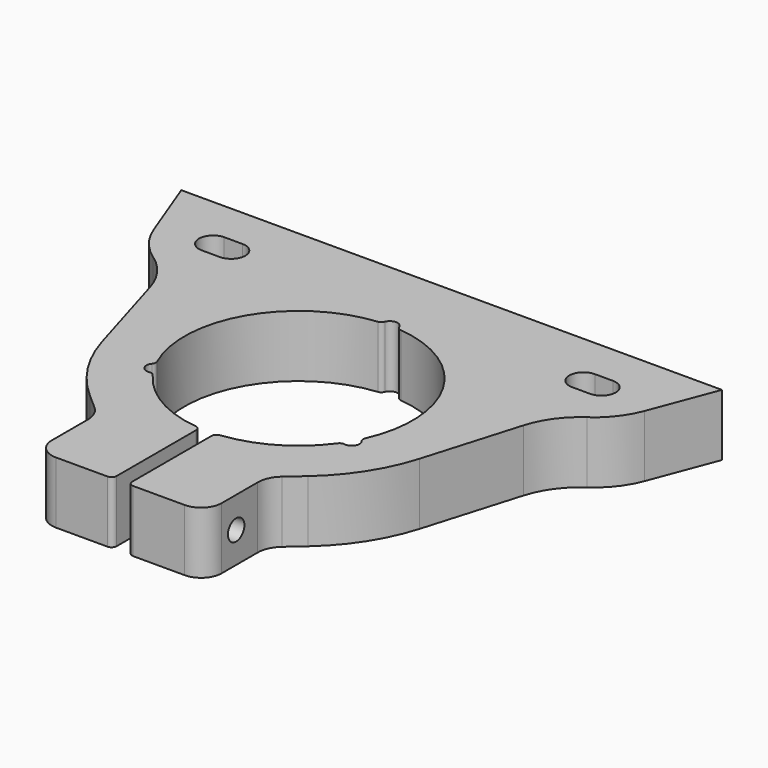
from build123d import *

# Parameters (mm, degrees)
F1_DEPTH = 12
F2_R     = 5
F3_R     = 2
F4_DEPTH = 69.001
F5_R     = 4
F6_R     = 2
F7_DEPTH = 12
F8_R     = 1.5
F9_DEPTH = 25
F10_R    = 1


with BuildPart() as f1:
    # F0 (on Top) → F1 (new body)
    with BuildSketch(Plane.XY):
        with BuildLine():
            Line((52.5, 0), (-52.5, 0))
            Line((-52.5, 0), (-47.6682177495, -12.7529115916))
            ThreePointArc((-47.6682177495, -12.7529115916), (-45.4487126417, -16.689553935), (-42.1574376197, -19.7864660409))
            ThreePointArc((-42.1574376197, -19.7864660409), (-38.5340554499, -23.3236951077), (-36.2940938248, -27.8650010584))
            Line((-36.2940938248, -27.8650010584), (-30.8201520188, -46.3009960956))
            ThreePointArc((-30.8201520188, -46.3009960956), (-27.0602921577, -54.5098124511), (-21.1662026167, -61.3494703824))
            Line((-21.1662026167, -61.3494703824), (-16.5, -65.4307906954))
            Line((-16.5, -65.4307906954), (-16.5, -80.4307906954))
            Line((-16.5, -80.4307906954), (-1.5, -80.4307906954))
            Line((-1.5, -80.4307906954), (-1.5, -59.2491515674))
            ThreePointArc((-1.5, -59.2491515674), (0, -15), (1.5, -59.2491515674))
            Line((1.5, -59.2491515674), (1.5, -80.4307906954))
            Line((1.5, -80.4307906954), (16.5, -80.4307906954))
            Line((16.5, -80.4307906954), (16.5, -65.4307906954))
            Line((16.5, -65.4307906954), (21.1662026167, -61.3494703824))
            ThreePointArc((21.1662026167, -61.3494703824), (27.0602921577, -54.5098124511), (30.8201520188, -46.3009960956))
            Line((30.8201520188, -46.3009960956), (36.2940938248, -27.8650010584))
            ThreePointArc((36.2940938248, -27.8650010584), (38.5340554499, -23.3236951077), (42.1574376197, -19.7864660409))
            ThreePointArc((42.1574376197, -19.7864660409), (45.4487126417, -16.689553935), (47.6682177495, -12.7529115916))
            Line((47.6682177495, -12.7529115916), (52.5, 0))
        make_face()
        with BuildLine():
            Line((-34.2147789885, -13.5), (-37.6424851382, -13.5))
            ThreePointArc((-37.6424851382, -13.5), (-40.4638530749, -10.8213679366), (-37.7852210115, -8))
            Line((-37.7852210115, -8), (-34.2147789885, -8))
            ThreePointArc((-34.2147789885, -8), (-31.4647789885, -10.75), (-34.2147789885, -13.5))
        make_face(mode=Mode.SUBTRACT)
        with BuildLine():
            ThreePointArc((37.7852210115, -8), (40.4638530749, -10.8213679366), (37.6424851382, -13.5))
            Line((37.6424851382, -13.5), (34.2147789885, -13.5))
            ThreePointArc((34.2147789885, -13.5), (31.4647789885, -10.75), (34.2147789885, -8))
            Line((34.2147789885, -8), (37.7852210115, -8))
        make_face(mode=Mode.SUBTRACT)
    extrude(amount=F1_DEPTH)

    # F2
    f2_edges = [f1.edges().sort_by_distance(p)[0] for p in [
        (-16.5, -65.430791, 6),
        (16.5, -65.430791, 6),
    ]]
    fillet(f2_edges, radius=F2_R)

    # F3 (on face) → F4 (cut, through all)
    with BuildSketch(Plane(origin=(-16.5, 0, 0), x_dir=(0, -1, 0), z_dir=(-1, 0, 0))):
        with Locations((72.9307906954, 6)):
            Circle(F3_R)
    extrude(amount=-F4_DEPTH, mode=Mode.SUBTRACT)

    # F5
    f5_edges = [f1.edges().sort_by_distance(p)[0] for p in [
        (-16.5, -80.430791, 6),
        (16.5, -80.430791, 6),
    ]]
    fillet(f5_edges, radius=F5_R)

    # F6 (on face) → F7 (cut)
    with BuildSketch(Plane(origin=(0, 0, 0), x_dir=(-1, 0, 0), z_dir=(0, 1, 0))):
        with Locations((-36, 6)):
            Circle(F6_R)
        with Locations((36, 6)):
            Circle(F6_R)
    extrude(amount=-F7_DEPTH, mode=Mode.SUBTRACT)

    # F8 (on face) → F9 (cut)
    with BuildSketch(Plane.XY.offset(12)):
        with Locations((0, -15)):
            Circle(F8_R)
        with Locations((-19.1824626938, -48.225)):
            Circle(F8_R)
        with Locations((19.1824626938, -48.225)):
            Circle(F8_R)
    extrude(amount=-F9_DEPTH, mode=Mode.SUBTRACT)

    # F10
    f10_edges = [f1.edges().sort_by_distance(p)[0] for p in [
        (1.49914, -15.05079, 6),
        (-1.49914, -15.05079, 6),
        (-19.888047, -46.901312, 6),
        (-18.388907, -49.497898, 6),
        (18.388907, -49.497898, 6),
        (19.888047, -46.901312, 6),
        (1.5, -59.249152, 6),
        (-1.5, -59.249152, 6),
        (1.5, -80.430791, 6),
        (-1.5, -80.430791, 6),
    ]]
    fillet(f10_edges, radius=F10_R)


solid = f1.part
